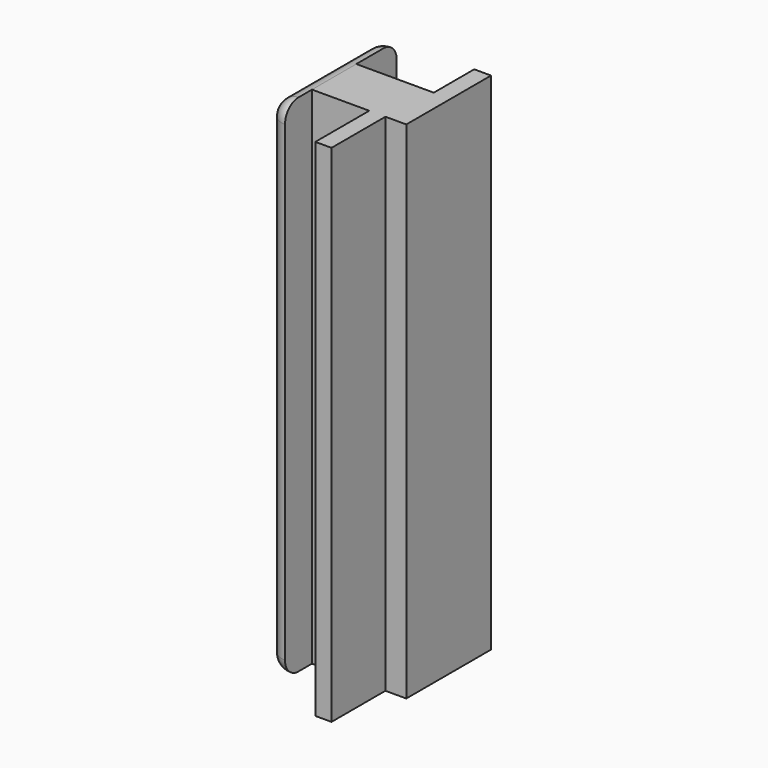
from build123d import *

# Parameters (mm, degrees)
F1_DEPTH = 150
F2_W     = 34.5892625776
F2_H     = 120
F3_DEPTH = 25
F4_R     = 4.99999


# Not quite as in the source:
# - a fillet or chamfer is up to 0.001 mm smaller than in the source, because OpenCascade refuses the exact size


with BuildPart() as f1:
    # F0 (on Top) → F1 (new body)
    with BuildSketch(Plane.XY):
        Polygon((-17, 31.4391109618), (-22, 31.4391109618), (-22, -10), (-17, -10), (-17, 0), (0, 0), (0, -20), (4.7985620563, -20), (4.7985620563, 0), (11, 0), (11, 31.4391109618), (6, 31.4391109618), (6, 16.4391109618), (-17, 16.4391109618), align=None)
    extrude(amount=F1_DEPTH)

    # F2 (on Right) → F3 (cut)
    with BuildSketch(Plane.YZ):
        with Locations((38.7337422506, 75)):
            Rectangle(F2_W, F2_H)
    extrude(amount=-F3_DEPTH, mode=Mode.SUBTRACT)

    # F4 (radius 5 in the source; OpenCascade refuses exactly that, so slightly less here)
    f4_edges = [f1.edges().sort_by_distance(p)[0] for p in [
        (-19.5, 21.439111, 135),
        (-19.5, 31.439111, 135),
        (-19.5, 21.439111, 15),
        (-19.5, 31.439111, 15),
        (-19.5, 31.439111, 150),
        (-19.5, -10, 150),
        (-19.5, 31.439111, 0),
        (-19.5, -10, 0),
        (-22, 10.719555, 0),
        (-22, -10, 75),
        (-22, 10.719555, 150),
        (-22, 31.439111, 142.5),
        (-22, 26.439111, 135),
        (-22, 21.439111, 75),
        (-22, 26.439111, 15),
        (-22, 31.439111, 7.5),
    ]]
    fillet(f4_edges, radius=F4_R)


solid = f1.part
